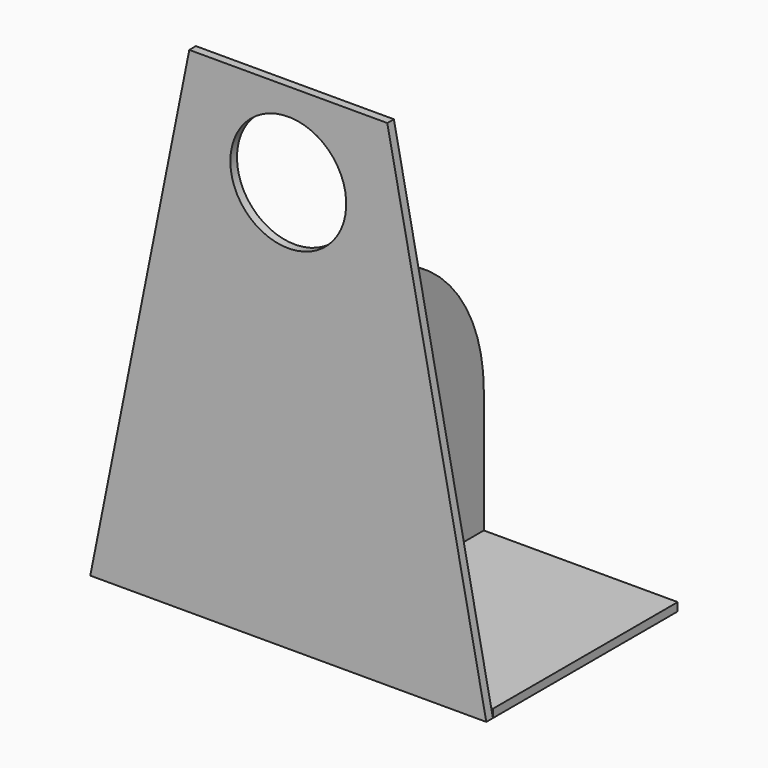
from build123d import *

# Parameters (mm, degrees)
F3_DEPTH = 6.35
F4_D     = 89.1794
F5_W     = 304.8
F5_H     = 177.8
F6_DEPTH = 6.35
F7_W     = 3.175
F7_H     = 221.1080746889
F8_DEPTH = 177.8
F9_R     = 127


# Not quite as in the source:
# - a variable given as a bare number and used for a length is read in inches; the dataset says mm whatever the document's units were


with BuildPart() as f3:
    # F1 (on Front) → F3 (new body)
    with BuildSketch(Plane.XZ):
        Polygon((129.7632297397, 381), (-22.6367702603, 381), (-98.8367702603, 0), (205.9632297397, 0), align=None)
    extrude(amount=F3_DEPTH)

    # F4 (through all)
    with Locations(Plane(origin=(0, 0, 0), x_dir=(1, 0, 0), z_dir=(0, 1, 0))):
        with Locations((53.5632297397, -315.9252)):
            Hole(F4_D / 2)

    # F5 (on Top) → F6 (join)
    with BuildSketch(Plane.XY):
        with Locations((53.5632297397, 88.9)):
            Rectangle(F5_W, F5_H)
    extrude(amount=F6_DEPTH)

    # F7 (on face) → F8 (join)
    with BuildSketch(Plane(origin=(0, 0, 0), x_dir=(-1, 0, 0), z_dir=(0, 1, 0))):
        with Locations((-55.1507297397, 116.9040373445)):
            Rectangle(F7_W, F7_H)
        with Locations((-51.9757297397, 116.9040373445)):
            Rectangle(F7_W, F7_H)
    extrude(amount=F8_DEPTH)

    # F9
    f9_edges = [f3.edges().sort_by_distance(p)[0] for p in [
        (53.56323, 177.8, 227.458075),
    ]]
    fillet(f9_edges, radius=F9_R)


solid = f3.part
